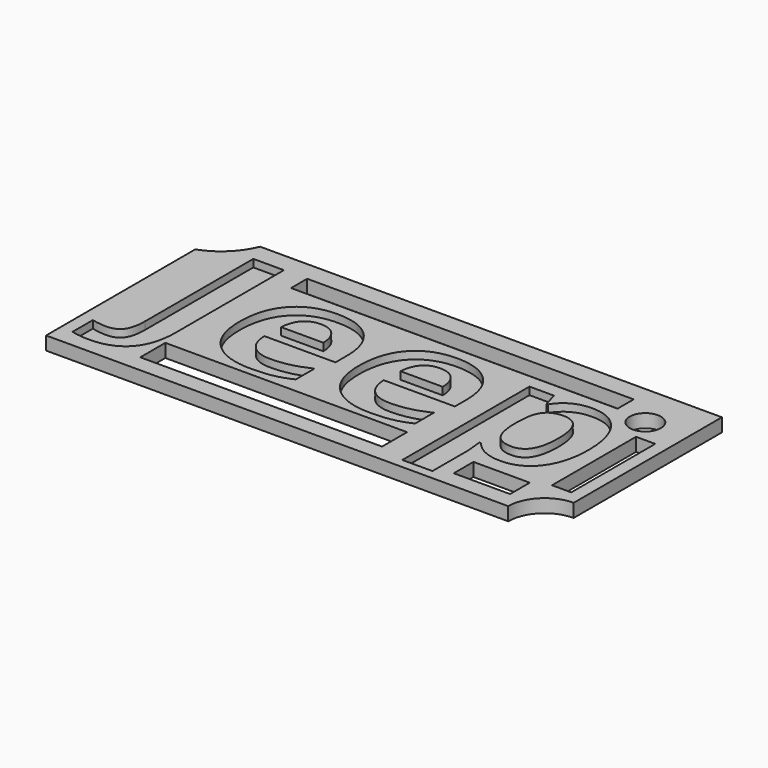
from build123d import *

# Parameters (mm, degrees)
F0_W         = 68.5800015926
F0_H         = 25.3263637424
F1_DEPTH     = 1.524
F2_TEXT_SIZE = 23.0909092352
F3_DEPTH     = 0.8636
F4_W         = 21.3907025754
F4_H         = 44.1902270541
F5_DEPTH     = 64.008
F6_R         = 1.7831774824
F7_DEPTH     = 17.5768
F8_R         = 7.1355221456
F9_DEPTH     = 58.674
F10_R        = 4.1556973334
F11_DEPTH    = 87.884
F12_W        = 27.623988688
F12_H        = 3.5755650606
F13_DEPTH    = 5.08
F14_W        = 37.3076461256
F14_H        = 2.303860656
F15_DEPTH    = 22.606
F16_W        = 2.195415087
F16_H        = 11.997720354
F17_DEPTH    = 13.462
F18_W        = 6.4349919558
F18_H        = 2.8093971778
F19_DEPTH    = 16.256


# Not quite as in the source:
# - Text() gives the source's letters only with a copy of the font that has no kerning and outlines rounded to 1/6400 em; it was checked with that copy


with BuildPart() as f1:
    # F0 (on Top) → F1 (new body)
    with BuildSketch(Plane.XY):
        with Locations((-34.2900007963, 12.6631818712)):
            Rectangle(F0_W, F0_H)
    extrude(amount=F1_DEPTH)

    # F2 (on face) → F3 (cut)
    with BuildSketch(Plane.XY.offset(1.524)):
        with Locations((-65.4627308249, 6.6227279603)):
            Text('Jeep', F2_TEXT_SIZE, font='Open Sans', font_style=FontStyle.BOLD, text_align=(TextAlign.LEFT, TextAlign.BOTTOM))
    extrude(amount=-F3_DEPTH, mode=Mode.SUBTRACT)

    # F4 (on face) → F5 (cut)
    with BuildSketch(Plane.XY.offset(1.524)):
        with Locations((-0.9227506816, 9.9933748133)):
            Rectangle(F4_W, F4_H)
    extrude(amount=-F5_DEPTH, mode=Mode.SUBTRACT)

    # F6 (on face) → F7 (cut)
    with BuildSketch(Plane.XY.offset(1.524)):
        with Locations((-16.3436960429, 20.291082561)):
            Circle(F6_R)
    extrude(amount=-F7_DEPTH, mode=Mode.SUBTRACT)

    # F8 (on face) → F9 (cut)
    with BuildSketch(Plane.XY.offset(1.524)):
        with Locations((-70.9923058748, 28.0106216669)):
            Circle(F8_R)
    extrude(amount=-F9_DEPTH, mode=Mode.SUBTRACT)

    # F10 (on face) → F11 (cut)
    with BuildSketch(Plane.XY.offset(1.524)):
        with Locations((-11.6181019694, 0)):
            Circle(F10_R)
    extrude(amount=-F11_DEPTH, mode=Mode.SUBTRACT)

    # F12 (on face) → F13 (cut)
    with BuildSketch(Plane.XY.offset(1.524)):
        with Locations((-45.5682575703, 3.7438283907)):
            Rectangle(F12_W, F12_H)
    extrude(amount=-F13_DEPTH, mode=Mode.SUBTRACT)

    # F14 (on face) → F15 (cut)
    with BuildSketch(Plane.XY.offset(1.524)):
        with Locations((-38.5805238038, 21.9555420535)):
            Rectangle(F14_W, F14_H)
    extrude(amount=-F15_DEPTH, mode=Mode.SUBTRACT)

    # F16 (on face) → F17 (cut)
    with BuildSketch(Plane.XY.offset(1.524)):
        with Locations((-14.1492676921, 11.5956576246)):
            Rectangle(F16_W, F16_H)
    extrude(amount=-F17_DEPTH, mode=Mode.SUBTRACT)

    # F18 (on face) → F19 (cut)
    with BuildSketch(Plane.XY.offset(1.524)):
        with Locations((-20.3258767724, 3.3377803629)):
            Rectangle(F18_W, F18_H)
    extrude(amount=-F19_DEPTH, mode=Mode.SUBTRACT)


solid = f1.part
